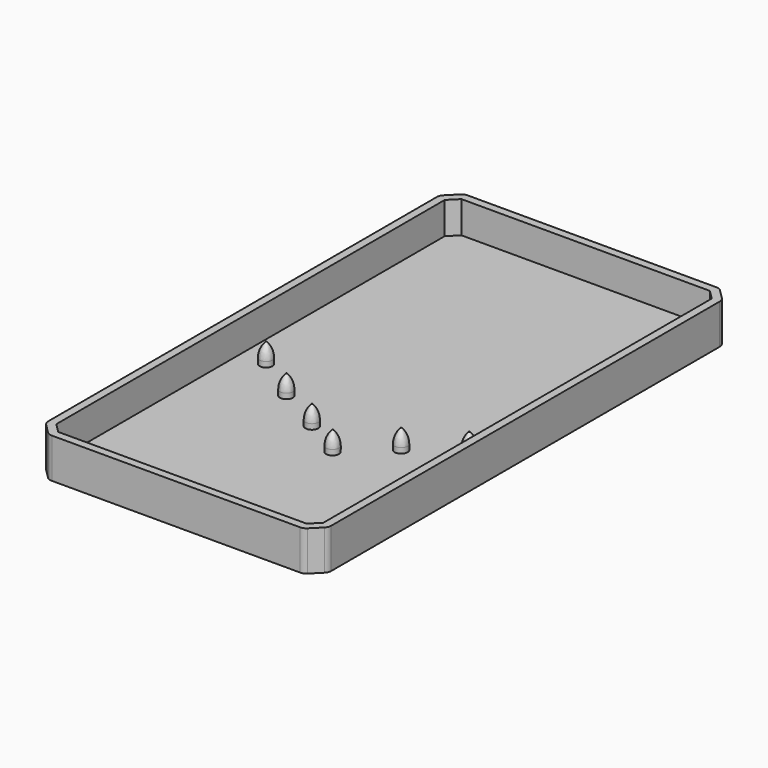
from build123d import *

# Parameters (mm, degrees)
F0_W     = 71
F0_H     = 130.5
F1_DEPTH = 10
F2_SIZE  = 3.5
F3_R     = 2
F4_T     = 2
F5_R     = 1.6
F6_DEPTH = 5
F7_SIZE  = 1.6
F8_R     = 5


# Not quite as in the source:
# - a shell that OpenCascade refuses in one call is made with other operations: the cavity is built on its own and cut out


with BuildPart() as f1:
    # F0 (on Top) → F1 (new body)
    with BuildSketch(Plane.XY):
        Rectangle(F0_W, F0_H)
    extrude(amount=F1_DEPTH)

    # F2
    f2_edges = [f1.edges().sort_by_distance(p)[0] for p in [
        (-35.5, -65.25, 5),
        (35.5, -65.25, 5),
        (-35.5, 65.25, 5),
        (35.5, 65.25, 5),
    ]]
    chamfer(f2_edges, length=F2_SIZE)

    # F3
    f3_edges = [f1.edges().sort_by_distance(p)[0] for p in [
        (-32, 65.25, 5),
        (-35.5, 61.75, 5),
        (32, 65.25, 5),
        (35.5, 61.75, 5),
        (32, -65.25, 5),
        (35.5, -61.75, 5),
        (-35.5, -61.75, 5),
        (-32, -65.25, 5),
    ]]
    fillet(f3_edges, radius=F3_R)

    # F4: shell of thickness 2, made by hand


with BuildPart() as f4_core1:
    # F4_t2: copy of F1
    add(f1.part)

    # the walls: a layer under each face that stays
    f4_faces = [f4_core1.faces().sort_by_distance(p)[0] for p in [
        (0, -65.25, 5),
        (0, 0, 0),
        (-33.75, -63.5, 5),
        (33.75, -63.5, 5),
        (-35.5, 0, 5),
        (35.5, 0, 5),
        (-33.75, 63.5, 5),
        (33.75, 63.5, 5),
        (0, 65.25, 5),
    ]]
    thicken(f4_faces, amount=-F4_T, mode=Mode.SUBTRACT)


with BuildPart() as f1_1:
    add(f1.part)

    # what is left inside the walls is the cavity
    f4_cavity = [f4_core1.part.solids().sort_by_distance(p)[0] for p in [
        (0, -21.083333, 2.02),
    ]]
    add(f4_cavity, mode=Mode.SUBTRACT)

    # F5 (on face) → F6 (join)
    with BuildSketch(Plane.XY.offset(2)):
        with Locations((-27, -3.25)):
            Circle(F5_R)
        with Locations((-15.5, -11.25)):
            Circle(F5_R)
        with Locations((-3.5, -18.25)):
            Circle(F5_R)
        with Locations((6.5, -24.25)):
            Circle(F5_R)
        with Locations((16.5, -15.25)):
            Circle(F5_R)
        with Locations((28, -8.25)):
            Circle(F5_R)
    extrude(amount=F6_DEPTH)

    # F7
    f7_edges = [f1_1.edges().sort_by_distance(p)[0] for p in [
        (-28.6, -3.25, 7),
        (-17.1, -11.25, 7),
        (-5.1, -18.25, 7),
        (4.9, -24.25, 7),
        (14.9, -15.25, 7),
        (26.4, -8.25, 7),
    ]]
    chamfer(f7_edges, length=F7_SIZE)

    # F8
    f8_edges = [f1_1.edges().sort_by_distance(p)[0] for p in [
        (-28.6, -3.25, 5.4),
        (-17.1, -11.25, 5.4),
        (-5.1, -18.25, 5.4),
        (4.9, -24.25, 5.4),
        (14.9, -15.25, 5.4),
        (26.4, -8.25, 5.4),
    ]]
    fillet(f8_edges, radius=F8_R)


solid = f1_1.part
